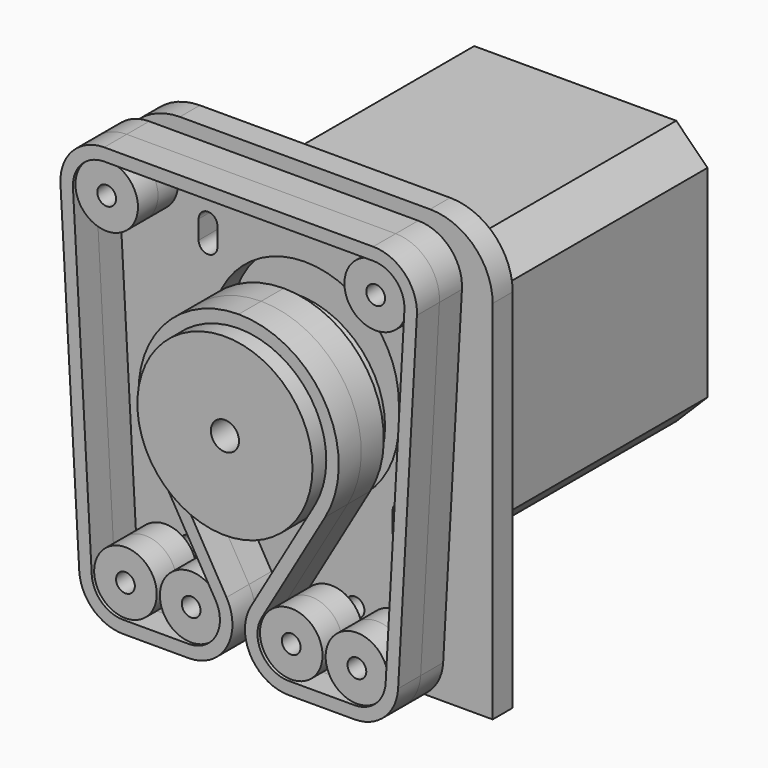
from build123d import *

# Parameters (mm, degrees)
F0_W      = 60
F0_H      = 68.5436762869
F0_R      = 1.5
F1_DEPTH  = 4
F2_W      = 42.3
F2_H      = 42.3
F3_DEPTH  = 50
F4_SIZE   = 5
F5_R      = 2.25
F6_DEPTH  = 15
F8_R      = 8
F8_R_2    = 2.25
F9_DEPTH  = 5.5
F10_R     = 14
F10_R_2   = 2.25
F11_DEPTH = 14.5
F13_R     = 5
F13_R_2   = 1.5
F14_DEPTH = 4
F15_DEPTH = 4
F17_DEPTH = 4.5
F18_R     = 10


with BuildPart() as f1:
    # F0 (on Front) → F1 (new body)
    with BuildSketch(Plane.XZ):
        with Locations((0, -2.3833755404)):
            Rectangle(F0_W, F0_H)
        with Locations((-18.5, -28)):
            Circle(F0_R, mode=Mode.SUBTRACT)
        with Locations((-8, -28)):
            Circle(F0_R, mode=Mode.SUBTRACT)
        with BuildLine():
            ThreePointArc((-17, -12.5), (-15.5, -11), (-14, -12.5))
            Line((-14, -12.5), (-14, -15.5))
            ThreePointArc((-14, -15.5), (-15.5, -17), (-17, -15.5))
            Line((-17, -15.5), (-17, -12.5))
        make_face(mode=Mode.SUBTRACT)
        with Locations((8, -28)):
            Circle(F0_R, mode=Mode.SUBTRACT)
        with Locations((18.5, -28)):
            Circle(F0_R, mode=Mode.SUBTRACT)
        with BuildLine():
            Line((14, -15.5), (14, -12.5))
            ThreePointArc((14, -12.5), (15.5, -11), (17, -12.5))
            Line((17, -12.5), (17, -15.5))
            ThreePointArc((17, -15.5), (15.5, -17), (14, -15.5))
        make_face(mode=Mode.SUBTRACT)
        with BuildLine():
            ThreePointArc((-17, 18.5), (-15.5, 20), (-14, 18.5))
            Line((-14, 18.5), (-14, 15.5))
            ThreePointArc((-14, 15.5), (-15.5, 14), (-17, 15.5))
            Line((-17, 15.5), (-17, 18.5))
        make_face(mode=Mode.SUBTRACT)
        with Locations((-21.5, 25.5)):
            Circle(F0_R, mode=Mode.SUBTRACT)
        with BuildLine():
            ThreePointArc((15, 0), (0, -15), (-15, 0))
            Line((-15, 0), (-15, 3))
            ThreePointArc((-15, 3), (0, 18), (15, 3))
            Line((15, 3), (15, 0))
        make_face(mode=Mode.SUBTRACT)
        with BuildLine():
            Line((17, 18.5), (17, 15.5))
            ThreePointArc((17, 15.5), (15.5, 14), (14, 15.5))
            Line((14, 15.5), (14, 18.5))
            ThreePointArc((14, 18.5), (15.5, 20), (17, 18.5))
        make_face(mode=Mode.SUBTRACT)
        with Locations((21.5, 25.5)):
            Circle(F0_R, mode=Mode.SUBTRACT)
    extrude(amount=-F1_DEPTH)

    # F18
    f18_edges = [f1.edges().sort_by_distance(p)[0] for p in [
        (-30, 2, 31.888463),
        (30, 2, 31.888463),
    ]]
    fillet(f18_edges, radius=F18_R)


with BuildPart() as f3:
    # F2 (on face) → F3 (new body)
    with BuildSketch(Plane(origin=(0, 4, 0), x_dir=(-1, 0, 0), z_dir=(0, 1, 0))):
        Rectangle(F2_W, F2_H)
    extrude(amount=F3_DEPTH)

    # F4
    f4_edges = [f3.edges().sort_by_distance(p)[0] for p in [
        (-21.15, 29, 21.15),
        (21.15, 29, 21.15),
        (-21.15, 29, -21.15),
        (21.15, 29, -21.15),
    ]]
    chamfer(f4_edges, length=F4_SIZE)

    # F5 (on face) → F6 (join)
    with BuildSketch(Plane.XZ.offset(-4)):
        Circle(F5_R)
    extrude(amount=F6_DEPTH)


with BuildPart() as f9:
    # F8 (on offset) → F9 (new body)
    with BuildSketch(Plane.XZ.offset(-4)):
        Circle(F8_R)
        Circle(F8_R_2, mode=Mode.SUBTRACT)
    extrude(amount=F9_DEPTH)

    # F10 (on face) → F11 (join)
    with BuildSketch(Plane.XZ.offset(1.5)):
        Circle(F10_R)
        Circle(F10_R_2, mode=Mode.SUBTRACT)
    extrude(amount=F11_DEPTH)


with BuildPart() as f14:
    # F13 (on mid) → F14 (new body)
    with BuildSketch(Plane.XZ.offset(8.75)):
        with Locations((-18.5, -28)):
            Circle(F13_R)
        with Locations((-18.5, -28)):
            Circle(F13_R_2, mode=Mode.SUBTRACT)
    extrude(amount=F14_DEPTH)


with BuildPart() as f14b:
    # F13 (on mid) → F14, piece 2 (new body)
    with BuildSketch(Plane.XZ.offset(8.75)):
        with Locations((-8, -28)):
            Circle(F13_R)
        with Locations((-8, -28)):
            Circle(F13_R_2, mode=Mode.SUBTRACT)
    extrude(amount=F14_DEPTH)


with BuildPart() as f14c:
    # F13 (on mid) → F14, piece 3 (new body)
    with BuildSketch(Plane.XZ.offset(8.75)):
        with Locations((8, -28)):
            Circle(F13_R)
        with Locations((8, -28)):
            Circle(F13_R_2, mode=Mode.SUBTRACT)
    extrude(amount=F14_DEPTH)


with BuildPart() as f14d:
    # F13 (on mid) → F14, piece 4 (new body)
    with BuildSketch(Plane.XZ.offset(8.75)):
        with Locations((18.5, -28)):
            Circle(F13_R)
        with Locations((18.5, -28)):
            Circle(F13_R_2, mode=Mode.SUBTRACT)
    extrude(amount=F14_DEPTH)


with BuildPart() as f14e:
    # F13 (on mid) → F14, piece 5 (new body)
    with BuildSketch(Plane.XZ.offset(8.75)):
        with Locations((-21.5, 25.5)):
            Circle(F13_R)
        with Locations((-21.5, 25.5)):
            Circle(F13_R_2, mode=Mode.SUBTRACT)
    extrude(amount=F14_DEPTH)


with BuildPart() as f14f:
    # F13 (on mid) → F14, piece 6 (new body)
    with BuildSketch(Plane.XZ.offset(8.75)):
        with Locations((21.5, 25.5)):
            Circle(F13_R)
        with Locations((21.5, 25.5)):
            Circle(F13_R_2, mode=Mode.SUBTRACT)
    extrude(amount=F14_DEPTH)


with BuildPart() as f15:
    # F15 (new): a face of the model
    f15_faces = [f14d.part.faces().sort_by_distance(p)[0] for p in [
        (13.6414213562, -8.75, -28),
    ]]
    extrude(f15_faces, amount=F15_DEPTH)


with BuildPart() as f15b:
    # F15#2 (new): a face of the model
    f15_2_faces = [f14c.part.faces().sort_by_distance(p)[0] for p in [
        (3.1414213562, -8.75, -28),
    ]]
    extrude(f15_2_faces, amount=F15_DEPTH)


with BuildPart() as f15c:
    # F15#3 (new): a face of the model
    f15_3_faces = [f14b.part.faces().sort_by_distance(p)[0] for p in [
        (-12.8585786438, -8.75, -28),
    ]]
    extrude(f15_3_faces, amount=F15_DEPTH)


with BuildPart() as f15d:
    # F15#4 (new): a face of the model
    f15_4_faces = [f14.part.faces().sort_by_distance(p)[0] for p in [
        (-23.3585786438, -8.75, -28),
    ]]
    extrude(f15_4_faces, amount=F15_DEPTH)


with BuildPart() as f15e:
    # F15#5 (new): a face of the model
    f15_5_faces = [f14e.part.faces().sort_by_distance(p)[0] for p in [
        (-26.3585786438, -8.75, 25.5),
    ]]
    extrude(f15_5_faces, amount=F15_DEPTH)


with BuildPart() as f15f:
    # F15#6 (new): a face of the model
    f15_6_faces = [f14f.part.faces().sort_by_distance(p)[0] for p in [
        (16.6414213562, -8.75, 25.5),
    ]]
    extrude(f15_6_faces, amount=F15_DEPTH)


with BuildPart() as f17:
    # F16 (on mid) → F17 (new body, symmetric)
    with BuildSketch(Plane.XZ.offset(8.75)):
        with BuildLine():
            ThreePointArc((0, 14), (12.1367694801, 6.9784544554), (12.0994132933, -7.0430247733))
            Line((12.0994132933, -7.0430247733), (1.9502933534, -24.4784876133))
            ThreePointArc((1.9502933534, -24.4784876133), (1.9316152599, -31.4892272277), (8, -35))
            Line((8, -35), (18.5, -35))
            ThreePointArc((18.5, -35), (23.3091915192, -33.0864208371), (25.4890205579, -28.3919076948))
            Line((25.4890205579, -28.3919076948), (28.4890205579, 25.1080923052))
            ThreePointArc((28.4890205579, 25.1080923052), (26.5864208371, 30.3091915192), (21.5, 32.5))
            Line((21.5, 32.5), (0, 32.5))
            Line((0, 32.5), (-21.5, 32.5))
            ThreePointArc((-21.5, 32.5), (-26.5864208371, 30.3091915192), (-28.4890205579, 25.1080923052))
            Line((-28.4890205579, 25.1080923052), (-25.4890205579, -28.3919076948))
            ThreePointArc((-25.4890205579, -28.3919076948), (-23.3091915192, -33.0864208371), (-18.5, -35))
            Line((-18.5, -35), (-8, -35))
            ThreePointArc((-8, -35), (-1.9316152599, -31.4892272277), (-1.9502933534, -24.4784876133))
            Line((-1.9502933534, -24.4784876133), (-12.0994132933, -7.0430247733))
            ThreePointArc((-12.0994132933, -7.0430247733), (-12.1367694801, 6.9784544554), (0, 14))
        make_face()
        with BuildLine():
            Line((18.5, -33), (8, -33))
            ThreePointArc((8, -33), (3.6654394714, -30.4923051627), (3.6787809667, -25.4846340095))
            Line((3.6787809667, -25.4846340095), (13.8279009066, -8.0491711695))
            ThreePointArc((13.8279009066, -8.0491711695), (13.8705936916, 7.9753765205), (0, 16))
            ThreePointArc((0, 16), (-13.8705936916, 7.9753765205), (-13.8279009066, -8.0491711695))
            Line((-13.8279009066, -8.0491711695), (-3.6787809667, -25.4846340095))
            ThreePointArc((-3.6787809667, -25.4846340095), (-3.6654394714, -30.4923051627), (-8, -33))
            Line((-8, -33), (-18.5, -33))
            ThreePointArc((-18.5, -33), (-21.9351367994, -31.6331577408), (-23.4921575414, -28.2799340677))
            Line((-23.4921575414, -28.2799340677), (-26.4921575414, 25.2200659323))
            ThreePointArc((-26.4921575414, 25.2200659323), (-25.1331577408, 28.9351367994), (-21.5, 30.5))
            Line((-21.5, 30.5), (0, 30.5))
            Line((0, 30.5), (21.5, 30.5))
            ThreePointArc((21.5, 30.5), (25.1331577408, 28.9351367994), (26.4921575414, 25.2200659323))
            Line((26.4921575414, 25.2200659323), (23.4921575414, -28.2799340677))
            ThreePointArc((23.4921575414, -28.2799340677), (21.9351367994, -31.6331577408), (18.5, -33))
        make_face(mode=Mode.SUBTRACT)
    extrude(amount=F17_DEPTH, both=True)


solid = Compound([f1.part, f3.part, f9.part, f14.part, f14b.part, f14c.part, f14d.part, f14e.part, f14f.part, f15.part, f15b.part, f15c.part, f15d.part, f15e.part, f15f.part, f17.part])
